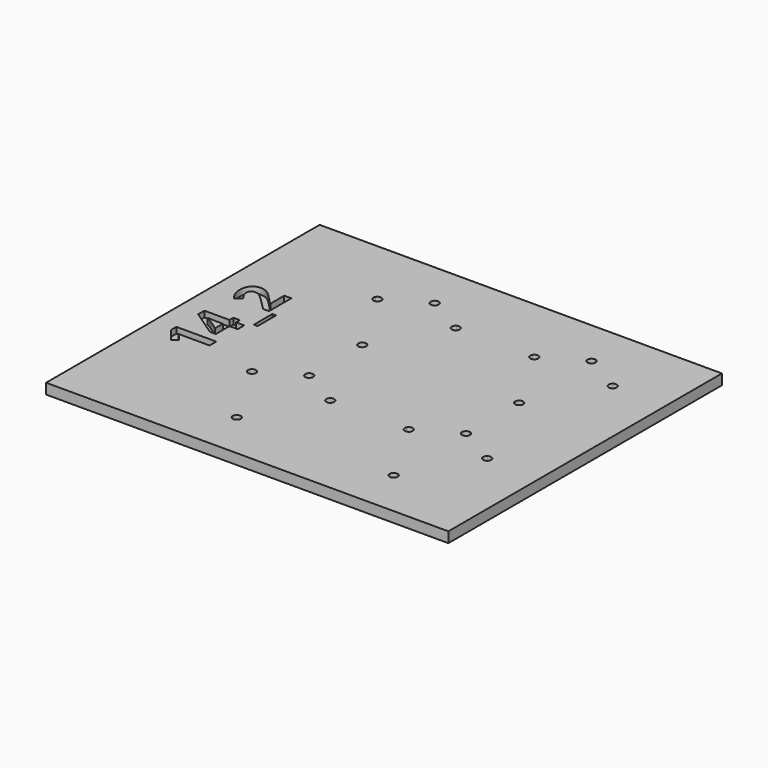
from build123d import *

# Parameters (mm, degrees)
F0_W         = 100
F0_H         = 85
F1_DEPTH     = 2.6
F2_TEXT_SIZE = 13.8888888889
F3_DEPTH     = 1.5
F5_DEPTH     = 2.6


# Not quite as in the source:
# - Text() gives the source's letters only with a copy of the font that has no kerning and outlines rounded to 1/6400 em; it was checked with that copy


with BuildPart() as f1:
    # F0 (on Top) → F1 (new body)
    with BuildSketch(Plane.XY):
        with Locations((6.8412768841, 20.8350909071)):
            Rectangle(F0_W, F0_H)
    extrude(amount=F1_DEPTH)

    # F2 (on face) → F3 (cut)
    with BuildSketch(Plane.XY.offset(2.6)):
        with Locations(Location((-28.1587231159, 6.7350909071), (0, 0, 90))):
            Text('14_2', F2_TEXT_SIZE, font='Open Sans', font_style=FontStyle.BOLD, text_align=(TextAlign.LEFT, TextAlign.BOTTOM))
    extrude(amount=-F3_DEPTH, mode=Mode.SUBTRACT)

    # F4 (on face) → F5 (cut, through all)
    with BuildSketch(Plane.XY.offset(2.6)):
        with BuildLine():
            ThreePointArc((-14.3635129618, 46.8030383321), (-15.1387936852, 46.9315310415), (-15.7675343123, 46.4600909071))
            Line((-15.7675343123, 46.4600909071), (-14.9015089085, 45.9600909071))
            ThreePointArc((-14.9015089085, 45.9600909071), (-14.6418816475, 46.3875453072), (-14.3635129618, 46.8030383321))
        make_face()
        with BuildLine():
            ThreePointArc((-14.3635129618, 46.8030383321), (-14.6418816475, 46.3875453072), (-14.9015089085, 45.9600909071))
            Line((-14.9015089085, 45.9600909071), (-14.0354835047, 45.4600909071))
            ThreePointArc((-14.0354835047, 45.4600909071), (-13.9355830822, 45.701271862), (-13.9015089085, 45.9600909071))
            ThreePointArc((-13.9015089085, 45.9600909071), (-14.0245836133, 46.440717609), (-14.3635129618, 46.8030383321))
        make_face()
        with BuildLine():
            Line((-14.0354835047, 45.4600909071), (-14.9015089085, 45.9600909071))
            ThreePointArc((-14.9015089085, 45.9600909071), (-15.1418816475, 45.5215199034), (-15.3625248193, 45.0726990376))
            ThreePointArc((-15.3625248193, 45.0726990376), (-14.6212834859, 45.000156684), (-14.0354835047, 45.4600909071))
        make_face()
        with BuildLine():
            Line((-14.9015089085, 45.9600909071), (-15.7675343123, 46.4600909071))
            ThreePointArc((-15.7675343123, 46.4600909071), (-15.8614431315, 45.6798654844), (-15.3625248193, 45.0726990376))
            ThreePointArc((-15.3625248193, 45.0726990376), (-15.1418816475, 45.5215199034), (-14.9015089085, 45.9600909071))
        make_face()
        with BuildLine():
            Line((-5.1587231159, 51.5850909071), (-5.1587231159, 52.5850909071))
            ThreePointArc((-5.1587231159, 52.5850909071), (-5.8813725622, 52.2763056188), (-6.1577349734, 51.5406464626))
            ThreePointArc((-6.1577349734, 51.5406464626), (-5.6587231159, 51.5739743035), (-5.1587231159, 51.5850909071))
        make_face()
        with BuildLine():
            ThreePointArc((-4.1587231159, 51.5850909071), (-4.4516163347, 52.2921976882), (-5.1587231159, 52.5850909071))
            Line((-5.1587231159, 52.5850909071), (-5.1587231159, 51.5850909071))
            ThreePointArc((-5.1587231159, 51.5850909071), (-4.6587231159, 51.5739743035), (-4.1597112585, 51.5406464626))
            ThreePointArc((-4.1597112585, 51.5406464626), (-4.1589701821, 51.5628631931), (-4.1587231159, 51.5850909071))
        make_face()
        with BuildLine():
            ThreePointArc((-4.1597112585, 51.5406464626), (-4.6587231159, 51.5739743035), (-5.1587231159, 51.5850909071))
            Line((-5.1587231159, 51.5850909071), (-5.1587231159, 50.5850909071))
            ThreePointArc((-5.1587231159, 50.5850909071), (-4.4675084041, 50.8624414608), (-4.1597112585, 51.5406464626))
        make_face()
        with BuildLine():
            Line((-5.1587231159, 50.5850909071), (-5.1587231159, 51.5850909071))
            ThreePointArc((-5.1587231159, 51.5850909071), (-5.6587231159, 51.5739743035), (-6.1577349734, 51.5406464626))
            ThreePointArc((-6.1577349734, 51.5406464626), (-5.8499378277, 50.8624414608), (-5.1587231159, 50.5850909071))
        make_face()
        with BuildLine():
            ThreePointArc((5.5840626767, 45.9600909071), (5.5499885029, 46.2189099522), (5.4500880804, 46.4600909071))
            Line((5.4500880804, 46.4600909071), (4.5840626767, 45.9600909071))
            ThreePointArc((4.5840626767, 45.9600909071), (4.8244354156, 45.5215199034), (5.0450785874, 45.0726990376))
            ThreePointArc((5.0450785874, 45.0726990376), (5.4387602579, 45.4409646752), (5.5840626767, 45.9600909071))
        make_face()
        with BuildLine():
            Line((3.7180372729, 45.4600909071), (4.5840626767, 45.9600909071))
            ThreePointArc((4.5840626767, 45.9600909071), (4.3244354156, 46.3875453072), (4.04606673, 46.8030383321))
            ThreePointArc((4.04606673, 46.8030383321), (3.6126225422, 46.1973756838), (3.7180372729, 45.4600909071))
        make_face()
        with BuildLine():
            Line((4.5840626767, 45.9600909071), (5.4500880804, 46.4600909071))
            ThreePointArc((5.4500880804, 46.4600909071), (4.8213474534, 46.9315310415), (4.04606673, 46.8030383321))
            ThreePointArc((4.04606673, 46.8030383321), (4.3244354156, 46.3875453072), (4.5840626767, 45.9600909071))
        make_face()
        with BuildLine():
            ThreePointArc((5.0450785874, 45.0726990376), (4.8244354156, 45.5215199034), (4.5840626767, 45.9600909071))
            Line((4.5840626767, 45.9600909071), (3.7180372729, 45.4600909071))
            ThreePointArc((3.7180372729, 45.4600909071), (4.303837254, 45.000156684), (5.0450785874, 45.0726990376))
        make_face()
        with BuildLine():
            Line((24.0984910915, 45.9600909071), (23.2324656877, 46.4600909071))
            ThreePointArc((23.2324656877, 46.4600909071), (23.1385568685, 45.6798654844), (23.6374751807, 45.0726990376))
            ThreePointArc((23.6374751807, 45.0726990376), (23.8581183525, 45.5215199034), (24.0984910915, 45.9600909071))
        make_face()
        with BuildLine():
            Line((24.9645164953, 45.4600909071), (24.0984910915, 45.9600909071))
            ThreePointArc((24.0984910915, 45.9600909071), (23.8581183525, 45.5215199034), (23.6374751807, 45.0726990376))
            ThreePointArc((23.6374751807, 45.0726990376), (24.3787165141, 45.000156684), (24.9645164953, 45.4600909071))
        make_face()
        with BuildLine():
            ThreePointArc((24.6364870382, 46.8030383321), (23.8612063148, 46.9315310415), (23.2324656877, 46.4600909071))
            Line((23.2324656877, 46.4600909071), (24.0984910915, 45.9600909071))
            ThreePointArc((24.0984910915, 45.9600909071), (24.3581183525, 46.3875453072), (24.6364870382, 46.8030383321))
        make_face()
        with BuildLine():
            ThreePointArc((24.6364870382, 46.8030383321), (24.3581183525, 46.3875453072), (24.0984910915, 45.9600909071))
            Line((24.0984910915, 45.9600909071), (24.9645164953, 45.4600909071))
            ThreePointArc((24.9645164953, 45.4600909071), (25.0644169178, 45.701271862), (25.0984910915, 45.9600909071))
            ThreePointArc((25.0984910915, 45.9600909071), (24.9754163867, 46.440717609), (24.6364870382, 46.8030383321))
        make_face()
        with BuildLine():
            ThreePointArc((34.8402887415, 51.5406464626), (34.3412768841, 51.5739743035), (33.8412768841, 51.5850909071))
            Line((33.8412768841, 51.5850909071), (33.8412768841, 50.5850909071))
            ThreePointArc((33.8412768841, 50.5850909071), (34.5324915959, 50.8624414608), (34.8402887415, 51.5406464626))
        make_face()
        with BuildLine():
            ThreePointArc((34.8412768841, 51.5850909071), (34.5483836653, 52.2921976882), (33.8412768841, 52.5850909071))
            Line((33.8412768841, 52.5850909071), (33.8412768841, 51.5850909071))
            ThreePointArc((33.8412768841, 51.5850909071), (34.3412768841, 51.5739743035), (34.8402887415, 51.5406464626))
            ThreePointArc((34.8402887415, 51.5406464626), (34.8410298179, 51.5628631931), (34.8412768841, 51.5850909071))
        make_face()
        with BuildLine():
            Line((33.8412768841, 50.5850909071), (33.8412768841, 51.5850909071))
            ThreePointArc((33.8412768841, 51.5850909071), (33.3412768841, 51.5739743035), (32.8422650266, 51.5406464626))
            ThreePointArc((32.8422650266, 51.5406464626), (33.1500621723, 50.8624414608), (33.8412768841, 50.5850909071))
        make_face()
        with BuildLine():
            Line((33.8412768841, 51.5850909071), (33.8412768841, 52.5850909071))
            ThreePointArc((33.8412768841, 52.5850909071), (33.1186274378, 52.2763056188), (32.8422650266, 51.5406464626))
            ThreePointArc((32.8422650266, 51.5406464626), (33.3412768841, 51.5739743035), (33.8412768841, 51.5850909071))
        make_face()
        with BuildLine():
            ThreePointArc((44.0450785874, 45.0726990376), (43.8244354156, 45.5215199034), (43.5840626767, 45.9600909071))
            Line((43.5840626767, 45.9600909071), (42.7180372729, 45.4600909071))
            ThreePointArc((42.7180372729, 45.4600909071), (43.303837254, 45.000156684), (44.0450785874, 45.0726990376))
        make_face()
        with BuildLine():
            Line((43.5840626767, 45.9600909071), (44.4500880804, 46.4600909071))
            ThreePointArc((44.4500880804, 46.4600909071), (43.8213474534, 46.9315310415), (43.04606673, 46.8030383321))
            ThreePointArc((43.04606673, 46.8030383321), (43.3244354156, 46.3875453072), (43.5840626767, 45.9600909071))
        make_face()
        with BuildLine():
            ThreePointArc((44.5840626767, 45.9600909071), (44.5499885029, 46.2189099522), (44.4500880804, 46.4600909071))
            Line((44.4500880804, 46.4600909071), (43.5840626767, 45.9600909071))
            ThreePointArc((43.5840626767, 45.9600909071), (43.8244354156, 45.5215199034), (44.0450785874, 45.0726990376))
            ThreePointArc((44.0450785874, 45.0726990376), (44.4387602579, 45.4409646752), (44.5840626767, 45.9600909071))
        make_face()
        with BuildLine():
            Line((42.7180372729, 45.4600909071), (43.5840626767, 45.9600909071))
            ThreePointArc((43.5840626767, 45.9600909071), (43.3244354156, 46.3875453072), (43.04606673, 46.8030383321))
            ThreePointArc((43.04606673, 46.8030383321), (42.6126225422, 46.1973756838), (42.7180372729, 45.4600909071))
        make_face()
        with BuildLine():
            ThreePointArc((-6.1577349734, 29.1295353515), (-5.6587231159, 29.0962075106), (-5.1587231159, 29.0850909071))
            Line((-5.1587231159, 29.0850909071), (-5.1587231159, 30.0850909071))
            ThreePointArc((-5.1587231159, 30.0850909071), (-5.8499378277, 29.8077403533), (-6.1577349734, 29.1295353515))
        make_face()
        with BuildLine():
            ThreePointArc((-6.1577349734, 29.1295353515), (-5.8813725622, 28.3938761953), (-5.1587231159, 28.0850909071))
            Line((-5.1587231159, 28.0850909071), (-5.1587231159, 29.0850909071))
            ThreePointArc((-5.1587231159, 29.0850909071), (-5.6587231159, 29.0962075106), (-6.1577349734, 29.1295353515))
        make_face()
        with BuildLine():
            Line((-5.1587231159, 29.0850909071), (-5.1587231159, 28.0850909071))
            ThreePointArc((-5.1587231159, 28.0850909071), (-4.4516163347, 28.3779841259), (-4.1587231159, 29.0850909071))
            ThreePointArc((-4.1587231159, 29.0850909071), (-4.1589701821, 29.107318621), (-4.1597112585, 29.1295353515))
            ThreePointArc((-4.1597112585, 29.1295353515), (-4.6587231159, 29.0962075106), (-5.1587231159, 29.0850909071))
        make_face()
        with BuildLine():
            Line((-5.1587231159, 30.0850909071), (-5.1587231159, 29.0850909071))
            ThreePointArc((-5.1587231159, 29.0850909071), (-4.6587231159, 29.0962075106), (-4.1597112585, 29.1295353515))
            ThreePointArc((-4.1597112585, 29.1295353515), (-4.4675084041, 29.8077403533), (-5.1587231159, 30.0850909071))
        make_face()
        with BuildLine():
            ThreePointArc((32.8422650266, 29.1295353515), (33.3412768841, 29.0962075106), (33.8412768841, 29.0850909071))
            Line((33.8412768841, 29.0850909071), (33.8412768841, 30.0850909071))
            ThreePointArc((33.8412768841, 30.0850909071), (33.1500621723, 29.8077403533), (32.8422650266, 29.1295353515))
        make_face()
        with BuildLine():
            ThreePointArc((32.8422650266, 29.1295353515), (33.1186274378, 28.3938761953), (33.8412768841, 28.0850909071))
            Line((33.8412768841, 28.0850909071), (33.8412768841, 29.0850909071))
            ThreePointArc((33.8412768841, 29.0850909071), (33.3412768841, 29.0962075106), (32.8422650266, 29.1295353515))
        make_face()
        with BuildLine():
            Line((33.8412768841, 29.0850909071), (33.8412768841, 28.0850909071))
            ThreePointArc((33.8412768841, 28.0850909071), (34.5483836653, 28.3779841259), (34.8412768841, 29.0850909071))
            ThreePointArc((34.8412768841, 29.0850909071), (34.8410298179, 29.107318621), (34.8402887415, 29.1295353515))
            ThreePointArc((34.8402887415, 29.1295353515), (34.3412768841, 29.0962075106), (33.8412768841, 29.0850909071))
        make_face()
        with BuildLine():
            Line((33.8412768841, 30.0850909071), (33.8412768841, 29.0850909071))
            ThreePointArc((33.8412768841, 29.0850909071), (34.3412768841, 29.0962075106), (34.8402887415, 29.1295353515))
            ThreePointArc((34.8402887415, 29.1295353515), (34.5324915959, 29.8077403533), (33.8412768841, 30.0850909071))
        make_face()
        with BuildLine():
            Line((-14.0354835047, 6.4600909071), (-14.9015089085, 6.9600909071))
            ThreePointArc((-14.9015089085, 6.9600909071), (-15.1418816475, 6.5215199034), (-15.3625248193, 6.0726990376))
            ThreePointArc((-15.3625248193, 6.0726990376), (-14.6212834859, 6.000156684), (-14.0354835047, 6.4600909071))
        make_face()
        with BuildLine():
            ThreePointArc((-14.3635129618, 7.8030383321), (-14.6418816475, 7.3875453072), (-14.9015089085, 6.9600909071))
            Line((-14.9015089085, 6.9600909071), (-14.0354835047, 6.4600909071))
            ThreePointArc((-14.0354835047, 6.4600909071), (-13.9355830822, 6.701271862), (-13.9015089085, 6.9600909071))
            ThreePointArc((-13.9015089085, 6.9600909071), (-14.0245836133, 7.440717609), (-14.3635129618, 7.8030383321))
        make_face()
        with BuildLine():
            Line((-14.9015089085, 6.9600909071), (-15.7675343123, 7.4600909071))
            ThreePointArc((-15.7675343123, 7.4600909071), (-15.8614431315, 6.6798654844), (-15.3625248193, 6.0726990376))
            ThreePointArc((-15.3625248193, 6.0726990376), (-15.1418816475, 6.5215199034), (-14.9015089085, 6.9600909071))
        make_face()
        with BuildLine():
            ThreePointArc((-14.3635129618, 7.8030383321), (-15.1387936852, 7.9315310415), (-15.7675343123, 7.4600909071))
            Line((-15.7675343123, 7.4600909071), (-14.9015089085, 6.9600909071))
            ThreePointArc((-14.9015089085, 6.9600909071), (-14.6418816475, 7.3875453072), (-14.3635129618, 7.8030383321))
        make_face()
        with BuildLine():
            ThreePointArc((5.5840626767, 6.9600909071), (5.5499885029, 7.2189099522), (5.4500880804, 7.4600909071))
            Line((5.4500880804, 7.4600909071), (4.5840626767, 6.9600909071))
            ThreePointArc((4.5840626767, 6.9600909071), (4.8244354156, 6.5215199034), (5.0450785874, 6.0726990376))
            ThreePointArc((5.0450785874, 6.0726990376), (5.4387602579, 6.4409646752), (5.5840626767, 6.9600909071))
        make_face()
        with BuildLine():
            Line((4.5840626767, 6.9600909071), (5.4500880804, 7.4600909071))
            ThreePointArc((5.4500880804, 7.4600909071), (4.8213474534, 7.9315310415), (4.04606673, 7.8030383321))
            ThreePointArc((4.04606673, 7.8030383321), (4.3244354156, 7.3875453072), (4.5840626767, 6.9600909071))
        make_face()
        with BuildLine():
            Line((3.7180372729, 6.4600909071), (4.5840626767, 6.9600909071))
            ThreePointArc((4.5840626767, 6.9600909071), (4.3244354156, 7.3875453072), (4.04606673, 7.8030383321))
            ThreePointArc((4.04606673, 7.8030383321), (3.6126225422, 7.1973756838), (3.7180372729, 6.4600909071))
        make_face()
        with BuildLine():
            ThreePointArc((5.0450785874, 6.0726990376), (4.8244354156, 6.5215199034), (4.5840626767, 6.9600909071))
            Line((4.5840626767, 6.9600909071), (3.7180372729, 6.4600909071))
            ThreePointArc((3.7180372729, 6.4600909071), (4.303837254, 6.000156684), (5.0450785874, 6.0726990376))
        make_face()
        with BuildLine():
            ThreePointArc((-4.1597112585, 12.5406464626), (-4.6587231159, 12.5739743035), (-5.1587231159, 12.5850909071))
            Line((-5.1587231159, 12.5850909071), (-5.1587231159, 11.5850909071))
            ThreePointArc((-5.1587231159, 11.5850909071), (-4.4675084041, 11.8624414608), (-4.1597112585, 12.5406464626))
        make_face()
        with BuildLine():
            Line((-5.1587231159, 11.5850909071), (-5.1587231159, 12.5850909071))
            ThreePointArc((-5.1587231159, 12.5850909071), (-5.6587231159, 12.5739743035), (-6.1577349734, 12.5406464626))
            ThreePointArc((-6.1577349734, 12.5406464626), (-5.8499378277, 11.8624414608), (-5.1587231159, 11.5850909071))
        make_face()
        with BuildLine():
            ThreePointArc((-4.1587231159, 12.5850909071), (-4.4516163347, 13.2921976882), (-5.1587231159, 13.5850909071))
            Line((-5.1587231159, 13.5850909071), (-5.1587231159, 12.5850909071))
            ThreePointArc((-5.1587231159, 12.5850909071), (-4.6587231159, 12.5739743035), (-4.1597112585, 12.5406464626))
            ThreePointArc((-4.1597112585, 12.5406464626), (-4.1589701821, 12.5628631931), (-4.1587231159, 12.5850909071))
        make_face()
        with BuildLine():
            Line((-5.1587231159, 12.5850909071), (-5.1587231159, 13.5850909071))
            ThreePointArc((-5.1587231159, 13.5850909071), (-5.8813725622, 13.2763056188), (-6.1577349734, 12.5406464626))
            ThreePointArc((-6.1577349734, 12.5406464626), (-5.6587231159, 12.5739743035), (-5.1587231159, 12.5850909071))
        make_face()
        with BuildLine():
            ThreePointArc((24.6364870382, 7.8030383321), (23.8612063148, 7.9315310415), (23.2324656877, 7.4600909071))
            Line((23.2324656877, 7.4600909071), (24.0984910915, 6.9600909071))
            ThreePointArc((24.0984910915, 6.9600909071), (24.3581183525, 7.3875453072), (24.6364870382, 7.8030383321))
        make_face()
        with BuildLine():
            ThreePointArc((24.6364870382, 7.8030383321), (24.3581183525, 7.3875453072), (24.0984910915, 6.9600909071))
            Line((24.0984910915, 6.9600909071), (24.9645164953, 6.4600909071))
            ThreePointArc((24.9645164953, 6.4600909071), (25.0644169178, 6.701271862), (25.0984910915, 6.9600909071))
            ThreePointArc((25.0984910915, 6.9600909071), (24.9754163867, 7.440717609), (24.6364870382, 7.8030383321))
        make_face()
        with BuildLine():
            Line((43.5840626767, 6.9600909071), (44.4500880804, 7.4600909071))
            ThreePointArc((44.4500880804, 7.4600909071), (43.8213474534, 7.9315310415), (43.04606673, 7.8030383321))
            ThreePointArc((43.04606673, 7.8030383321), (43.3244354156, 7.3875453072), (43.5840626767, 6.9600909071))
        make_face()
        with BuildLine():
            ThreePointArc((44.5840626767, 6.9600909071), (44.5499885029, 7.2189099522), (44.4500880804, 7.4600909071))
            Line((44.4500880804, 7.4600909071), (43.5840626767, 6.9600909071))
            ThreePointArc((43.5840626767, 6.9600909071), (43.8244354156, 6.5215199034), (44.0450785874, 6.0726990376))
            ThreePointArc((44.0450785874, 6.0726990376), (44.4387602579, 6.4409646752), (44.5840626767, 6.9600909071))
        make_face()
        with BuildLine():
            ThreePointArc((44.0450785874, 6.0726990376), (43.8244354156, 6.5215199034), (43.5840626767, 6.9600909071))
            Line((43.5840626767, 6.9600909071), (42.7180372729, 6.4600909071))
            ThreePointArc((42.7180372729, 6.4600909071), (43.303837254, 6.000156684), (44.0450785874, 6.0726990376))
        make_face()
        with BuildLine():
            Line((24.9645164953, 6.4600909071), (24.0984910915, 6.9600909071))
            ThreePointArc((24.0984910915, 6.9600909071), (23.8581183525, 6.5215199034), (23.6374751807, 6.0726990376))
            ThreePointArc((23.6374751807, 6.0726990376), (24.3787165141, 6.000156684), (24.9645164953, 6.4600909071))
        make_face()
        with BuildLine():
            Line((24.0984910915, 6.9600909071), (23.2324656877, 7.4600909071))
            ThreePointArc((23.2324656877, 7.4600909071), (23.1385568685, 6.6798654844), (23.6374751807, 6.0726990376))
            ThreePointArc((23.6374751807, 6.0726990376), (23.8581183525, 6.5215199034), (24.0984910915, 6.9600909071))
        make_face()
        with BuildLine():
            Line((42.7180372729, 6.4600909071), (43.5840626767, 6.9600909071))
            ThreePointArc((43.5840626767, 6.9600909071), (43.3244354156, 7.3875453072), (43.04606673, 7.8030383321))
            ThreePointArc((43.04606673, 7.8030383321), (42.6126225422, 7.1973756838), (42.7180372729, 6.4600909071))
        make_face()
        with BuildLine():
            Line((33.8412768841, 12.5850909071), (33.8412768841, 13.5850909071))
            ThreePointArc((33.8412768841, 13.5850909071), (33.1186274378, 13.2763056188), (32.8422650266, 12.5406464626))
            ThreePointArc((32.8422650266, 12.5406464626), (33.3412768841, 12.5739743035), (33.8412768841, 12.5850909071))
        make_face()
        with BuildLine():
            Line((33.8412768841, 11.5850909071), (33.8412768841, 12.5850909071))
            ThreePointArc((33.8412768841, 12.5850909071), (33.3412768841, 12.5739743035), (32.8422650266, 12.5406464626))
            ThreePointArc((32.8422650266, 12.5406464626), (33.1500621723, 11.8624414608), (33.8412768841, 11.5850909071))
        make_face()
        with BuildLine():
            ThreePointArc((34.8412768841, 12.5850909071), (34.5483836653, 13.2921976882), (33.8412768841, 13.5850909071))
            Line((33.8412768841, 13.5850909071), (33.8412768841, 12.5850909071))
            ThreePointArc((33.8412768841, 12.5850909071), (34.3412768841, 12.5739743035), (34.8402887415, 12.5406464626))
            ThreePointArc((34.8402887415, 12.5406464626), (34.8410298179, 12.5628631931), (34.8412768841, 12.5850909071))
        make_face()
        with BuildLine():
            ThreePointArc((34.8402887415, 12.5406464626), (34.3412768841, 12.5739743035), (33.8412768841, 12.5850909071))
            Line((33.8412768841, 12.5850909071), (33.8412768841, 11.5850909071))
            ThreePointArc((33.8412768841, 11.5850909071), (34.5324915959, 11.8624414608), (34.8402887415, 12.5406464626))
        make_face()
        with BuildLine():
            Line((-5.1587231159, -9.9149090929), (-5.1587231159, -10.9149090929))
            ThreePointArc((-5.1587231159, -10.9149090929), (-4.4516163347, -10.6220158741), (-4.1587231159, -9.9149090929))
            ThreePointArc((-4.1587231159, -9.9149090929), (-4.1589701821, -9.892681379), (-4.1597112585, -9.8704646485))
            ThreePointArc((-4.1597112585, -9.8704646485), (-4.6587231159, -9.9037924894), (-5.1587231159, -9.9149090929))
        make_face()
        with BuildLine():
            Line((-5.1587231159, -8.9149090929), (-5.1587231159, -9.9149090929))
            ThreePointArc((-5.1587231159, -9.9149090929), (-4.6587231159, -9.9037924894), (-4.1597112585, -9.8704646485))
            ThreePointArc((-4.1597112585, -9.8704646485), (-4.4675084041, -9.1922596467), (-5.1587231159, -8.9149090929))
        make_face()
        with BuildLine():
            ThreePointArc((-6.1577349734, -9.8704646485), (-5.6587231159, -9.9037924894), (-5.1587231159, -9.9149090929))
            Line((-5.1587231159, -9.9149090929), (-5.1587231159, -8.9149090929))
            ThreePointArc((-5.1587231159, -8.9149090929), (-5.8499378277, -9.1922596467), (-6.1577349734, -9.8704646485))
        make_face()
        with BuildLine():
            ThreePointArc((-6.1577349734, -9.8704646485), (-5.8813725622, -10.6061238047), (-5.1587231159, -10.9149090929))
            Line((-5.1587231159, -10.9149090929), (-5.1587231159, -9.9149090929))
            ThreePointArc((-5.1587231159, -9.9149090929), (-5.6587231159, -9.9037924894), (-6.1577349734, -9.8704646485))
        make_face()
        with BuildLine():
            Line((33.8412768841, -8.9149090929), (33.8412768841, -9.9149090929))
            ThreePointArc((33.8412768841, -9.9149090929), (34.3412768841, -9.9037924894), (34.8402887415, -9.8704646485))
            ThreePointArc((34.8402887415, -9.8704646485), (34.5324915959, -9.1922596467), (33.8412768841, -8.9149090929))
        make_face()
        with BuildLine():
            ThreePointArc((32.8422650266, -9.8704646485), (33.1186274378, -10.6061238047), (33.8412768841, -10.9149090929))
            Line((33.8412768841, -10.9149090929), (33.8412768841, -9.9149090929))
            ThreePointArc((33.8412768841, -9.9149090929), (33.3412768841, -9.9037924894), (32.8422650266, -9.8704646485))
        make_face()
        with BuildLine():
            ThreePointArc((32.8422650266, -9.8704646485), (33.3412768841, -9.9037924894), (33.8412768841, -9.9149090929))
            Line((33.8412768841, -9.9149090929), (33.8412768841, -8.9149090929))
            ThreePointArc((33.8412768841, -8.9149090929), (33.1500621723, -9.1922596467), (32.8422650266, -9.8704646485))
        make_face()
        with BuildLine():
            Line((33.8412768841, -9.9149090929), (33.8412768841, -10.9149090929))
            ThreePointArc((33.8412768841, -10.9149090929), (34.5483836653, -10.6220158741), (34.8412768841, -9.9149090929))
            ThreePointArc((34.8412768841, -9.9149090929), (34.8410298179, -9.892681379), (34.8402887415, -9.8704646485))
            ThreePointArc((34.8402887415, -9.8704646485), (34.3412768841, -9.9037924894), (33.8412768841, -9.9149090929))
        make_face()
    extrude(amount=-F5_DEPTH, mode=Mode.SUBTRACT)


solid = f1.part
